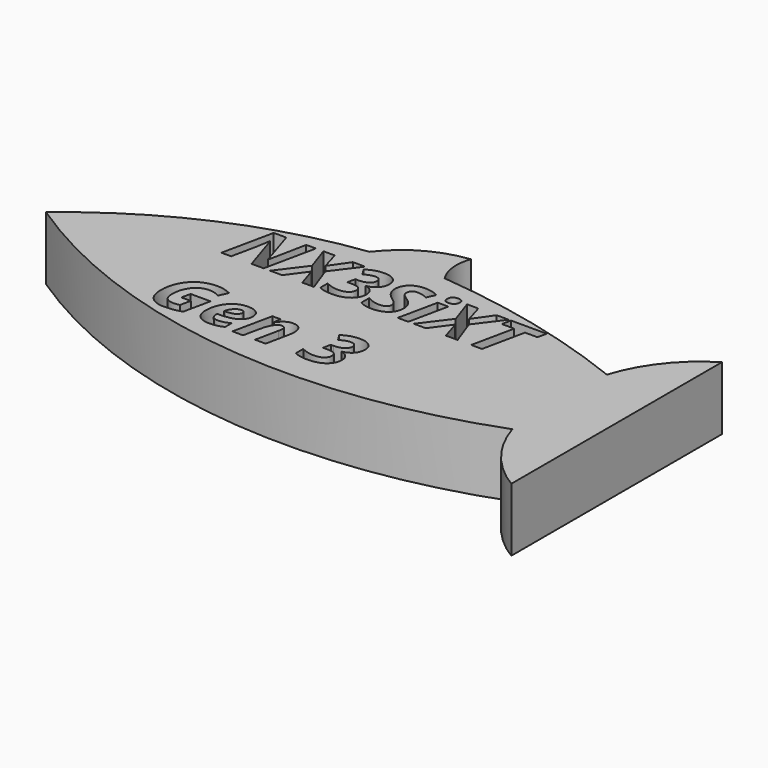
from build123d import *

# Parameters (mm, degrees)
F1_DEPTH     = 5
F2_TEXT_SIZE = 5.7127415795
F3_DEPTH     = 2


# Not quite as in the source:
# - Text() gives the source's letters only with a copy of the font that has no kerning and outlines rounded to 1/6400 em; it was checked with that copy


with BuildPart() as f1:
    # F0 (on Top) → F1 (new body)
    with BuildSketch(Plane.XY):
        with BuildLine():
            ThreePointArc((4.347845912, 11.4437388256), (1.2788254178, 10.4483783242), (-1.148430152, 8.3228055258))
            ThreePointArc((-1.148430152, 8.3228055258), (-11.1784422645, 5.5300074977), (-20, 0))
            ThreePointArc((-20, 0), (-0.3112886701, -7.2239189338), (20.5036979532, -4.6613634778))
            ThreePointArc((20.5036979532, -4.6613634778), (22.2303444484, -7.9323994631), (25, -10.383928101))
            Line((25, -10.383928101), (25, 0))
            Line((25, 0), (25, 10.383928101))
            ThreePointArc((25, 10.383928101), (22.2303444484, 7.9323994631), (20.5036979532, 4.6613634778))
            ThreePointArc((20.5036979532, 4.6613634778), (12.7240741405, 7.1175143829), (4.6757058026, 8.4513026094))
            ThreePointArc((4.6757058026, 8.4513026094), (4.1607154683, 9.9090575349), (4.347845912, 11.4437388256))
        make_face()
    extrude(amount=F1_DEPTH)

    # F2 (on face) → F3 (cut)
    with BuildSketch(Plane.XY.offset(5)):
        with Locations((-8.3415903792, 2.5292017106)):
            Text('NX3SiXT', F2_TEXT_SIZE, font='Open Sans', font_style=FontStyle.BOLDITALIC, text_align=(TextAlign.LEFT, TextAlign.BOTTOM))
        with Locations((-8.3415903792, -5.2401268376)):
            Text('Gen 3', F2_TEXT_SIZE, font='Open Sans', font_style=FontStyle.BOLDITALIC, text_align=(TextAlign.LEFT, TextAlign.BOTTOM))
    extrude(amount=-F3_DEPTH, mode=Mode.SUBTRACT)


solid = f1.part
